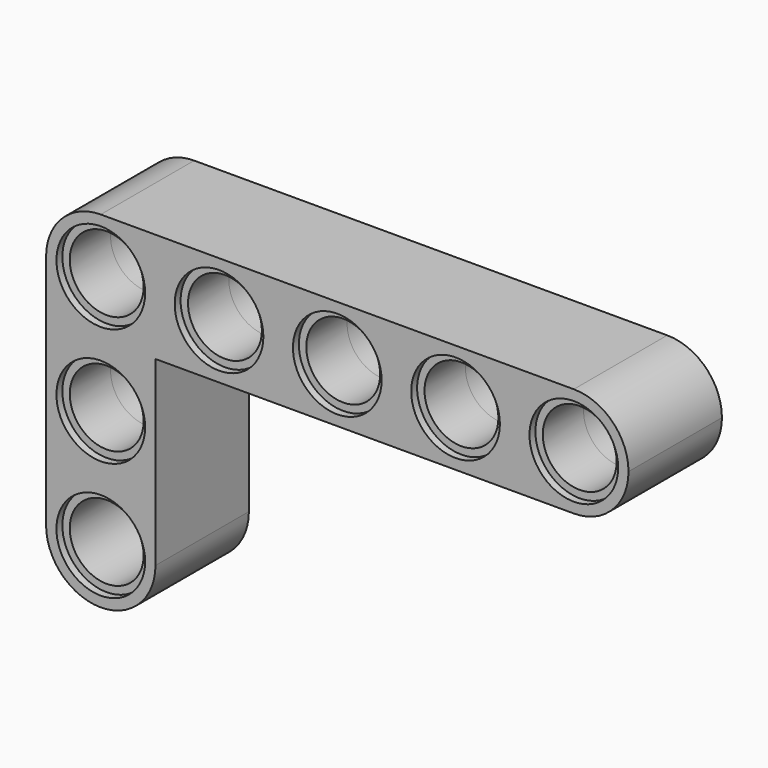
from build123d import *

# Parameters (mm, degrees)
F0_R     = 3
F1_DEPTH = 3.95
F0_R_2   = 2.499
F2_DEPTH = 3.45
F3_R     = 3.69999


# Not quite as in the source:
# - a fillet or chamfer is up to 0.001 mm smaller than in the source, because OpenCascade refuses the exact size


with BuildPart() as f1:
    # F0 (on Front) → F1 (new body, symmetric)
    with BuildSketch(Plane.XZ):
        Polygon((42.8304520275, -14.3135290742), (42.8304520275, -6.9135290742), (3.4304520275, -6.9135290742), (3.4304520275, -30.3135290742), (10.8304520275, -30.3135290742), (10.8304520275, -14.3135290742), align=None)
        with Locations((7.1304520275, -26.6135290742)):
            Circle(F0_R, mode=Mode.SUBTRACT)
        with Locations((7.1304520275, -18.6135290742)):
            Circle(F0_R, mode=Mode.SUBTRACT)
        with Locations((7.1304520275, -10.6135290742)):
            Circle(F0_R, mode=Mode.SUBTRACT)
        with Locations((15.1304520275, -10.6135290742)):
            Circle(F0_R, mode=Mode.SUBTRACT)
        with Locations((23.1304520275, -10.6135290742)):
            Circle(F0_R, mode=Mode.SUBTRACT)
        with Locations((31.1304520275, -10.6135290742)):
            Circle(F0_R, mode=Mode.SUBTRACT)
        with Locations((39.1304520275, -10.6135290742)):
            Circle(F0_R, mode=Mode.SUBTRACT)
    extrude(amount=F1_DEPTH, both=True)

    # F0 (on Front) → F2 (join, symmetric)
    with BuildSketch(Plane.XZ):
        with Locations((39.1304520275, -10.6135290742)):
            Circle(F0_R)
        with Locations((39.1304520275, -10.6135290742)):
            Circle(F0_R_2, mode=Mode.SUBTRACT)
        with Locations((31.1304520275, -10.6135290742)):
            Circle(F0_R)
        with Locations((31.1304520275, -10.6135290742)):
            Circle(F0_R_2, mode=Mode.SUBTRACT)
        with Locations((23.1304520275, -10.6135290742)):
            Circle(F0_R)
        with Locations((23.1304520275, -10.6135290742)):
            Circle(F0_R_2, mode=Mode.SUBTRACT)
        with Locations((15.1304520275, -10.6135290742)):
            Circle(F0_R)
        with Locations((15.1304520275, -10.6135290742)):
            Circle(F0_R_2, mode=Mode.SUBTRACT)
        with Locations((7.1304520275, -10.6135290742)):
            Circle(F0_R)
        with Locations((7.1304520275, -10.6135290742)):
            Circle(F0_R_2, mode=Mode.SUBTRACT)
        with Locations((7.1304520275, -18.6135290742)):
            Circle(F0_R)
        with Locations((7.1304520275, -18.6135290742)):
            Circle(F0_R_2, mode=Mode.SUBTRACT)
        with Locations((7.1304520275, -26.6135290742)):
            Circle(F0_R)
        with Locations((7.1304520275, -26.6135290742)):
            Circle(F0_R_2, mode=Mode.SUBTRACT)
    extrude(amount=F2_DEPTH, both=True)

    # F3 (radius 3.7 in the source; OpenCascade refuses exactly that, so slightly less here)
    f3_edges = [f1.edges().sort_by_distance(p)[0] for p in [
        (42.830452, 0, -6.913529),
        (42.830452, 0, -14.313529),
        (10.830452, 0, -30.313529),
        (3.430452, 0, -30.313529),
        (3.430452, 0, -6.913529),
    ]]
    fillet(f3_edges, radius=F3_R)


solid = f1.part
